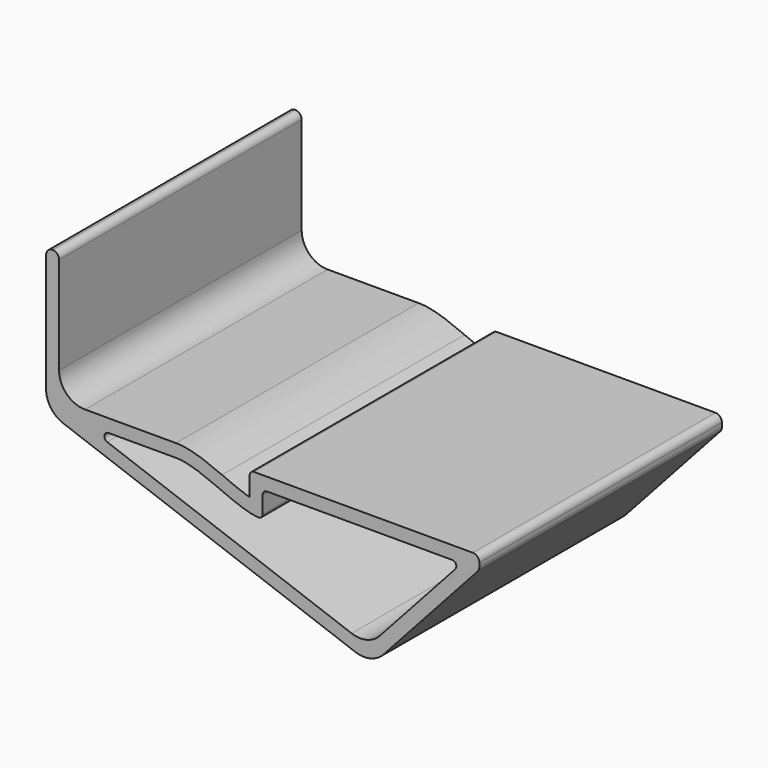
from build123d import *

# Parameters (mm, degrees)
F0_W         = 1.5
F0_H         = 15
F0_H_2       = 1.5
F1_DEPTH     = 35
F2_R         = 3
F3_R         = 0.5
F4_R         = 0.74999
F5_TEXT_SIZE = 7.8123211902
F6_DEPTH     = 0.4


# Not quite as in the source:
# - a fillet or chamfer is up to 0.001 mm smaller than in the source, because OpenCascade refuses the exact size
# - ends of sketch curves that miss each other by under 0.0002 mm in the source are joined
# - Text() gives the source's letters only with a copy of the font that has no kerning and outlines rounded to 1/6400 em; it was checked with that copy


with BuildPart() as f1:
    # F0 (on Front) → F1 (new body)
    with BuildSketch(Plane.XZ):
        with Locations((0.75, 9)):
            Rectangle(F0_W, F0_H)
        with BuildLine():
            Line((1.5, 1.5), (0, 1.5))
            Line((0, 1.5), (0, 0))
            Line((0, 0), (4.3857066002, 0))
            Line((4.3857066002, 0), (15, 0))
            Line((15, 0), (20.3076726165, 0))
            add(Edge.make_bspline(
                [(20.3076726165, 0), (19.9613391426, 0.1480763703), (19.1624921639, 0.4865686334), (17.8864112021, 0.9748848409), (16.4769611274, 1.3772161031), (15.5, 1.5), (15, 1.5)],
                knots=[0.5268596167, 0.5268596167, 0.5268596167, 0.5268596167, 0.625, 0.75, 0.875, 1, 1, 1, 1], degree=3))
            Line((15, 1.5), (1.5, 1.5))
        make_face()
        with BuildLine():
            add(Edge.make_bspline(
                [(23.5000271172, -1.2432669014), (23.3597225948, -1.2025116169), (22.8440957766, -1.0410149339), (21.8859439585, -0.6761057841), (20.9362434779, -0.2693177997), (20.4024591259, -0.0405263808), (20.3076726165, 0)],
                knots=[0.2014712136, 0.2014712136, 0.2014712136, 0.2014712136, 0.25, 0.375, 0.5, 0.5268596167, 0.5268596167, 0.5268596167, 0.5268596167], degree=3))
            Line((20.3076726165, 0), (15, 0))
            add(Edge.make_bspline(
                [(25, -3), (22, -3), (18, 0), (15, 0)],
                knots=[0, 0, 0, 0, 10.4403065089, 10.4403065089, 10.4403065089, 10.4403065089], degree=3))
            Line((25, -3), (25, 0))
            Line((25, 0), (23.5, 0))
            Line((23.5, 0), (23.5000271172, -1.2432669014))
        make_face()
        with Locations((24.25, 0.75)):
            Rectangle(F0_W, F0_H_2)
        Polygon((47.9746369682, 0), (50, 0), (50, 1.5), (25, 1.5), (25, 0), align=None)
        Polygon((38.1007350464, -12.2712668018), (37.5877048314, -13.680805733), (50, 0), (47.9746369682, 0), (37.153863572, -11.9266337695), align=None)
        Polygon((4.3857066002, 0), (0, 0), (37.5877048314, -13.680805733), (38.1007350464, -12.2712668018), (37.153863572, -11.9266337695), align=None)
    extrude(amount=F1_DEPTH)

    # F2
    f2_edges = [f1.edges().sort_by_distance(p)[0] for p in [
        (1.5, -17.5, 1.5),
        (0, -17.5, 0),
        (37.587705, -17.5, -13.680806),
        (37.153864, -17.5, -11.926634),
    ]]
    fillet(f2_edges, radius=F2_R)

    # F3
    f3_edges = [f1.edges().sort_by_distance(p)[0] for p in [
        (47.974637, -17.5, 0),
        (4.385707, -17.5, 0),
        (15, -17.5, 0),
        (23.5, -17.5, 1.5),
        (25, -17.5, 0),
        (25, -17.5, -3),
    ]]
    fillet(f3_edges, radius=F3_R)

    # F4 (radius 0.75 in the source; OpenCascade refuses exactly that, so slightly less here)
    f4_edges = [f1.edges().sort_by_distance(p)[0] for p in [
        (50, -17.5, 0),
        (50, -17.5, 1.5),
        (1.5, -17.5, 16.5),
        (0, -17.5, 16.5),
    ]]
    fillet(f4_edges, radius=F4_R)

    # F5 (on face) → F6 (cut)
    with BuildSketch(Plane(origin=(0, 0, 0), x_dir=(0.9396926208, 0, -0.3420201433), z_dir=(-0.3420201433, 0, -0.9396926208))):
        with Locations((4.0426717309, 14.6875643715)):
            Text('AIRSTER', F5_TEXT_SIZE, font='Open Sans', font_style=FontStyle.BOLD, text_align=(TextAlign.LEFT, TextAlign.BOTTOM))
    extrude(amount=-F6_DEPTH, mode=Mode.SUBTRACT)


solid = f1.part
